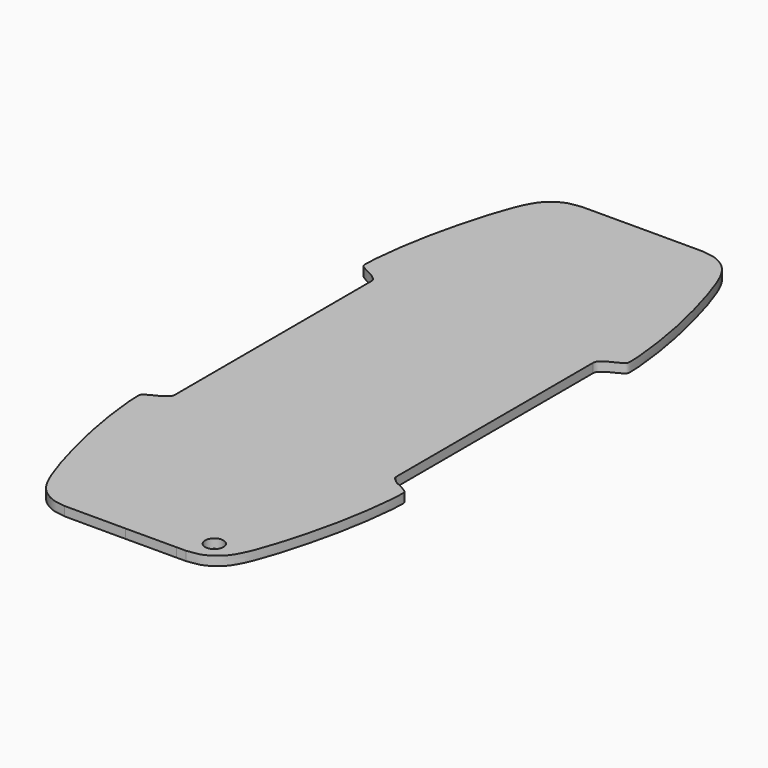
from build123d import *

# Parameters (mm, degrees)
F1_DEPTH = 0.5
F2_R     = 0.5
F3_DEPTH = 25


with BuildPart() as f1:
    # F0 (on Top) → F1 (new body)
    with BuildSketch(Plane.XY):
        with BuildLine():
            add(Edge.make_bspline(
                [(8.4428153932, 46.1577735841), (8.9348866368, 46.0957848403), (9.1902084572, 46.063620605), (10.2136533947, 45.482421242), (11.0515898848, 43.4474753339), (12.1103981, 39.4594863885), (12.4151111507, 36.3633669949), (12.340186084, 36.0679246479), (12.165975669, 35.9602462388), (11.9507020497, 35.8303573833), (11.6789376951, 35.7187516393), (11.4838684771, 35.6089894059), (11.2951492349, 35.402465646), (11.2299108219, 35.4186188516), (11.1919697374, 35.2088660002)],
                knots=[0, 0, 0, 0, 0.0587180961, 0.1205420114, 0.2138591133, 0.3506444227, 0.4605887666, 0.4905820957, 0.5177770546, 0.5504776042, 0.5852649664, 0.6163716927, 0.6468395023, 0.6799505505, 0.6799505505, 0.6799505505, 0.6799505505], degree=3))
            Line((8.4428153932, 46.1577735841), (7.9196737637, 46.1577735841))
            add(Edge.make_bspline(
                [(10.6898430557, 28.479457974), (10.2008874142, 35.3660491094), (9.3819124933, 45.0954346997), (7.9196737637, 46.1577735841)],
                knots=[0.7815795169, 0.7815795169, 0.7815795169, 0.7815795169, 0.988282322, 0.988282322, 0.988282322, 0.988282322], degree=3))
            add(Edge.make_bspline(
                [(11.1919697374, 35.2088660002), (11.0755157617, 34.5650638059), (10.9217010225, 31.865964087), (10.6898430557, 28.479457974)],
                knots=[0.6799505505, 0.6799505505, 0.6799505505, 0.6799505505, 0.7815795169, 0.7815795169, 0.7815795169, 0.7815795169], degree=3))
        make_face()
        with BuildLine():
            Line((11.2089504357, 21.7513385402), (11.1919697374, 35.2088660002))
            add(Edge.make_bspline(
                [(11.1919697374, 35.2088660002), (11.0755157617, 34.5650638059), (10.9217010225, 31.865964087), (10.6898430557, 28.479457974)],
                knots=[0.6799505505, 0.6799505505, 0.6799505505, 0.6799505505, 0.7815795169, 0.7815795169, 0.7815795169, 0.7815795169], degree=3))
            add(Edge.make_bspline(
                [(11.2089504357, 21.7513385402), (11.0908721351, 22.3948448019), (10.9302464525, 25.0935477601), (10.6898430557, 28.479457974)],
                knots=[0.6799505505, 0.6799505505, 0.6799505505, 0.6799505505, 0.7815795169, 0.7815795169, 0.7815795169, 0.7815795169], degree=3))
        make_face()
        with BuildLine():
            add(Edge.make_bspline(
                [(10.6898430557, 28.479457974), (10.2008874142, 35.3660491094), (9.3819124933, 45.0954346997), (7.9196737637, 46.1577735841)],
                knots=[0.7815795169, 0.7815795169, 0.7815795169, 0.7815795169, 0.988282322, 0.988282322, 0.988282322, 0.988282322], degree=3))
            Line((7.9196737637, 46.1577735841), (5.1296291058, 46.1577735841))
            Line((5.1296291058, 46.1577735841), (2.3395933321, 46.1507326427))
            add(Edge.make_bspline(
                [(-0.3859542385, 28.4654825411), (0.0856208824, 35.3532856734), (0.8800401713, 45.0847070435), (2.3395933321, 46.1507326427)],
                knots=[0.7815795169, 0.7815795169, 0.7815795169, 0.7815795169, 0.988282322, 0.988282322, 0.988282322, 0.988282322], degree=3))
            add(Edge.make_bspline(
                [(-0.3859542385, 28.4654825411), (0.103001403, 21.5788914057), (0.9219763239, 11.8495058153), (2.3842150534, 10.787166931)],
                knots=[0.7815795169, 0.7815795169, 0.7815795169, 0.7815795169, 0.988282322, 0.988282322, 0.988282322, 0.988282322], degree=3))
            Line((2.3842150534, 10.787166931), (5.1742597114, 10.787166931))
            Line((5.1742597114, 10.787166931), (7.9642954851, 10.7942078724))
            add(Edge.make_bspline(
                [(10.6898430557, 28.479457974), (10.2182679348, 21.5916548416), (9.4238486459, 11.8602334716), (7.9642954851, 10.7942078724)],
                knots=[0.7815795169, 0.7815795169, 0.7815795169, 0.7815795169, 0.988282322, 0.988282322, 0.988282322, 0.988282322], degree=3))
        make_face()
        with BuildLine():
            add(Edge.make_bspline(
                [(11.2089504357, 21.7513385402), (11.0908721351, 22.3948448019), (10.9302464525, 25.0935477601), (10.6898430557, 28.479457974)],
                knots=[0.6799505505, 0.6799505505, 0.6799505505, 0.6799505505, 0.7815795169, 0.7815795169, 0.7815795169, 0.7815795169], degree=3))
            add(Edge.make_bspline(
                [(10.6898430557, 28.479457974), (10.2182679348, 21.5916548416), (9.4238486459, 11.8602334716), (7.9642954851, 10.7942078724)],
                knots=[0.7815795169, 0.7815795169, 0.7815795169, 0.7815795169, 0.988282322, 0.988282322, 0.988282322, 0.988282322], degree=3))
            Line((7.9642954851, 10.7942078724), (8.4874354488, 10.7955280697))
            add(Edge.make_bspline(
                [(8.4874354488, 10.7955280697), (8.979348691, 10.8587584044), (9.2345885289, 10.8915668661), (10.2565634959, 11.4753471384), (11.0893619395, 13.5124011787), (12.1381027161, 17.5030494278), (12.4350014466, 20.5999279348), (12.3593310418, 20.8951802605), (12.1848494448, 21.0024186902), (11.9692487242, 21.1317638688), (11.6972035874, 21.2426834344), (11.5018579952, 21.3519530427), (11.3126181717, 21.5579998941), (11.2474207306, 21.5416821046), (11.2089504357, 21.7513385402)],
                knots=[0, 0, 0, 0, 0.0587180961, 0.1205420114, 0.2138591133, 0.3506444227, 0.4605887666, 0.4905820957, 0.5177770546, 0.5504776042, 0.5852649664, 0.6163716927, 0.6468395023, 0.6799505505, 0.6799505505, 0.6799505505, 0.6799505505], degree=3))
        make_face()
        with BuildLine():
            add(Edge.make_bspline(
                [(-0.3859542385, 28.4654825411), (0.0856208824, 35.3532856734), (0.8800401713, 45.0847070435), (2.3395933321, 46.1507326427)],
                knots=[0.7815795169, 0.7815795169, 0.7815795169, 0.7815795169, 0.988282322, 0.988282322, 0.988282322, 0.988282322], degree=3))
            Line((2.3395933321, 46.1507326427), (1.8164533684, 46.1494124454))
            add(Edge.make_bspline(
                [(1.8164533684, 46.1494124454), (1.3245401262, 46.0861821106), (1.0693002883, 46.053373649), (0.0473253212, 45.4695933766), (-0.7854731224, 43.4325393364), (-1.834213899, 39.4418910872), (-2.1311126294, 36.3450125803), (-2.0554422246, 36.0497602546), (-1.8809606277, 35.9425218249), (-1.6653599071, 35.8131766463), (-1.3933147702, 35.7022570807), (-1.197969178, 35.5929874724), (-1.0087293545, 35.3869406209), (-0.9435319134, 35.4032584105), (-0.9050616186, 35.1936019748)],
                knots=[0, 0, 0, 0, 0.0587180961, 0.1205420114, 0.2138591133, 0.3506444227, 0.4605887666, 0.4905820957, 0.5177770546, 0.5504776042, 0.5852649664, 0.6163716927, 0.6468395023, 0.6799505505, 0.6799505505, 0.6799505505, 0.6799505505], degree=3))
            add(Edge.make_bspline(
                [(-0.9050616186, 35.1936019748), (-0.7869833179, 34.5500957132), (-0.6263576353, 31.851392755), (-0.3859542385, 28.4654825411)],
                knots=[0.6799505505, 0.6799505505, 0.6799505505, 0.6799505505, 0.7815795169, 0.7815795169, 0.7815795169, 0.7815795169], degree=3))
        make_face()
        with BuildLine():
            add(Edge.make_bspline(
                [(-0.8880809202, 21.7360745149), (-0.7716269445, 22.3798767092), (-0.6178122053, 25.0789764281), (-0.3859542385, 28.4654825411)],
                knots=[0.6799505505, 0.6799505505, 0.6799505505, 0.6799505505, 0.7815795169, 0.7815795169, 0.7815795169, 0.7815795169], degree=3))
            add(Edge.make_bspline(
                [(-0.9050616186, 35.1936019748), (-0.7869833179, 34.5500957132), (-0.6263576353, 31.851392755), (-0.3859542385, 28.4654825411)],
                knots=[0.6799505505, 0.6799505505, 0.6799505505, 0.6799505505, 0.7815795169, 0.7815795169, 0.7815795169, 0.7815795169], degree=3))
            Line((-0.9050616186, 35.1936019748), (-0.8880809202, 21.7360745149))
        make_face()
        with BuildLine():
            add(Edge.make_bspline(
                [(-0.3859542385, 28.4654825411), (0.103001403, 21.5788914057), (0.9219763239, 11.8495058153), (2.3842150534, 10.787166931)],
                knots=[0.7815795169, 0.7815795169, 0.7815795169, 0.7815795169, 0.988282322, 0.988282322, 0.988282322, 0.988282322], degree=3))
            add(Edge.make_bspline(
                [(-0.8880809202, 21.7360745149), (-0.7716269445, 22.3798767092), (-0.6178122053, 25.0789764281), (-0.3859542385, 28.4654825411)],
                knots=[0.6799505505, 0.6799505505, 0.6799505505, 0.6799505505, 0.7815795169, 0.7815795169, 0.7815795169, 0.7815795169], degree=3))
            add(Edge.make_bspline(
                [(1.861073424, 10.787166931), (1.3690021804, 10.8491556748), (1.11368036, 10.8813199101), (0.0902354225, 11.4625192731), (-0.7477010677, 13.4974651812), (-1.8065092829, 17.4854541266), (-2.1112223335, 20.5815735202), (-2.0362972668, 20.8770158672), (-1.8620868518, 20.9846942763), (-1.6468132325, 21.1145831317), (-1.375048878, 21.2261888758), (-1.1799796599, 21.3359511092), (-0.9912604178, 21.5424748691), (-0.9260220048, 21.5263216634), (-0.8880809202, 21.7360745149)],
                knots=[0, 0, 0, 0, 0.0587180961, 0.1205420114, 0.2138591133, 0.3506444227, 0.4605887666, 0.4905820957, 0.5177770546, 0.5504776042, 0.5852649664, 0.6163716927, 0.6468395023, 0.6799505505, 0.6799505505, 0.6799505505, 0.6799505505], degree=3))
            Line((1.861073424, 10.787166931), (2.3842150534, 10.787166931))
        make_face()
    extrude(amount=F1_DEPTH)

    # F2 (on face) → F3 (cut)
    with BuildSketch(Plane.XY.offset(0.5)):
        with Locations((9.0170297772, 12.0532298461)):
            Circle(F2_R)
    extrude(amount=-F3_DEPTH, mode=Mode.SUBTRACT)


solid = f1.part
